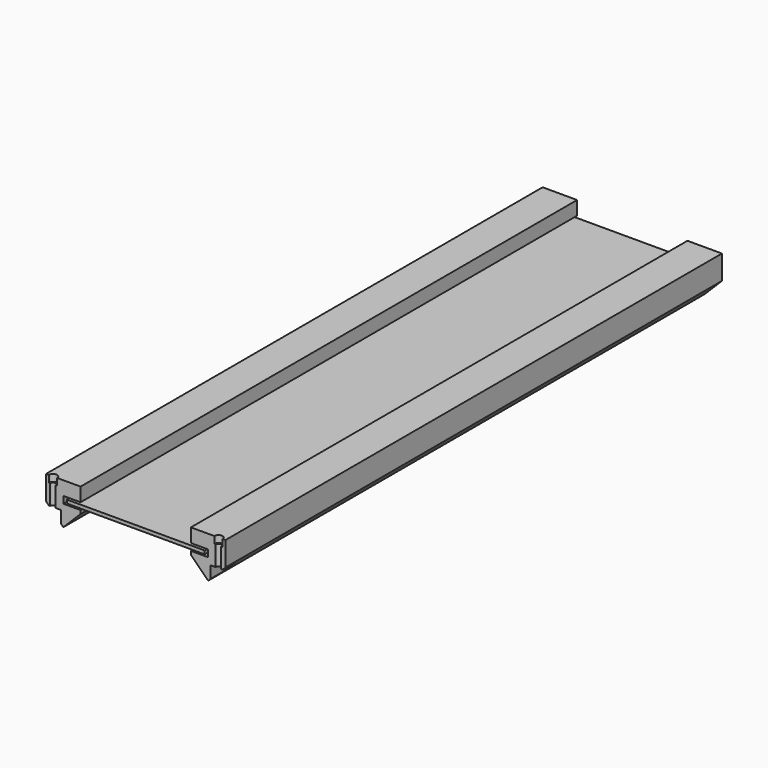
from build123d import *

# Parameters (mm, degrees)
F1_DEPTH      = 500
F2_W          = 100
F2_H          = 5
F3_DEPTH      = 500
F4_R          = 4
F6_DEPTH      = 60.001
F5_R          = 6
F7_DEPTH      = 10
F8_W          = 378.7088692188
F8_H          = 131.297647953
F9_DEPTH      = 60.001
F9_DEPTH_BACK = 1053
F11_DEPTH     = 25


# Not quite as in the source:
# - an extrude ends at something that could not be found from the text; its depth is read off the source's solid


with BuildPart() as f1:
    # F0 (on Front) → F1 (new body, symmetric)
    with BuildSketch(Plane.XZ):
        Polygon((50, 0), (0, 0), (0, -35), (25, -60), (50, -35), (50, -30), (25, -30), (25, -20), (50, -20), align=None)
    extrude(amount=F1_DEPTH, both=True)

    # F4 (on Top) → F6 (cut, through all)
    with BuildSketch(Plane.XY):
        with Locations((10, -400)):
            Circle(F4_R)
    extrude(amount=-F6_DEPTH, mode=Mode.SUBTRACT)

    # F5 (on Top) → F7 (cut)
    with BuildSketch(Plane.XY):
        with Locations((10, -400)):
            Circle(F5_R)
    extrude(amount=-F7_DEPTH, mode=Mode.SUBTRACT)


with BuildPart() as f3:
    # F2 (on Front) → F3 (new body, symmetric)
    with BuildSketch(Plane.XZ):
        with Locations((80, -25.5)):
            Rectangle(F2_W, F2_H)
    extrude(amount=F3_DEPTH, both=True)


with BuildPart() as f9_tool:
    # F8 (on Top) → F9 (new body, two sides)
    with BuildSketch(Plane.XY) as f9_sk:
        with Locations((61.5063756704, -465.6488239765)):
            Rectangle(F8_W, F8_H)
    extrude(amount=-F9_DEPTH)
    extrude(f9_sk.sketch, amount=F9_DEPTH_BACK)


with BuildPart() as f1_1:
    add(f1.part)

    # F9: cut by f9_tool
    add(f9_tool.part, mode=Mode.SUBTRACT)

    # F10 (on face) → F11 (cut)
    with BuildSketch(Plane.XZ.offset(400)):
        Polygon((14, -39.0548482537), (-6.0729645193, -39.0548482537), (-6.0729645193, -62.4141655862), (21.4163064957, -62.4141655862), (21.4163064957, -56.4163064957), (14, -49), align=None)
        Polygon((21.4163064957, -39.0548482537), (14, -39.0548482537), (14, -49), (21.4163064957, -56.4163064957), align=None)
    extrude(amount=-F11_DEPTH, mode=Mode.SUBTRACT)


with BuildPart() as f3_1:
    add(f3.part)

    # F9: cut by f9_tool
    add(f9_tool.part, mode=Mode.SUBTRACT)



with BuildPart() as f3_2:
    add(f3_1.part)
    # F12: F1, F3 across face
    add(f1_1.part.mirror(Plane(origin=(130, 50, -25.5), x_dir=(0, 1, 0), z_dir=(1, 0, 0))))
    add(f3_1.part.mirror(Plane(origin=(130, 50, -25.5), x_dir=(0, 1, 0), z_dir=(1, 0, 0))))


solid = Compound([f1_1.part, f3_2.part])
